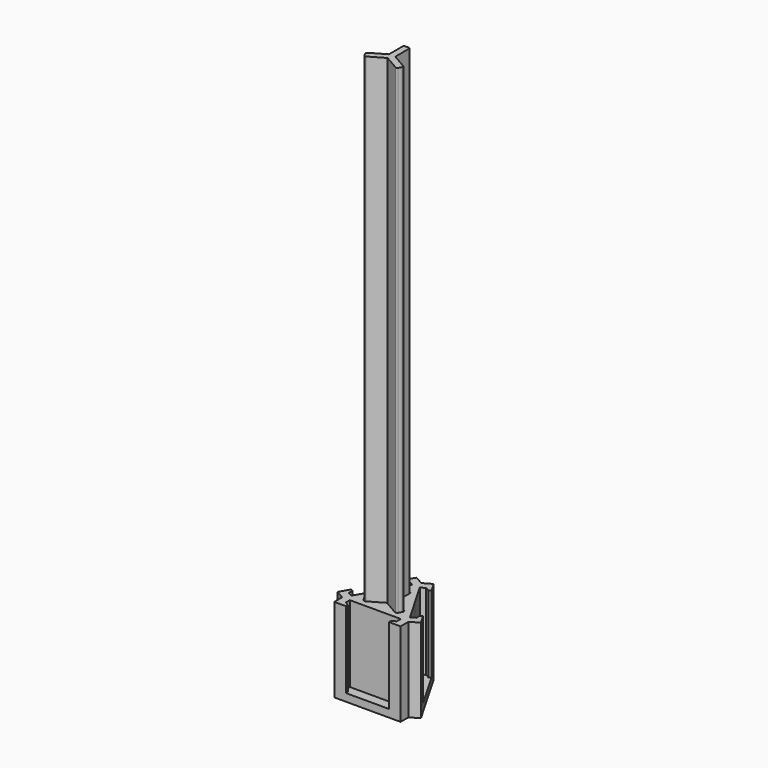
from build123d import *

# Parameters (mm, degrees)
F1_DEPTH      = 30
F3_DEPTH      = 3
F5_DEPTH      = 20
F5_DEPTH_BACK = 188
F6_OFFSET     = 0.3


with BuildPart() as f1:
    # F0 (on Top) → F1 (new body)
    with BuildSketch(Plane.XY):
        Polygon((-10, -7.5055534995), (0, -7.5055534995), (10, -7.5055534995), (10, -9.5055534995), (8.5, -10.3715789032), (8.5, -11.3715789032), (13, -11.3715789032), (13, -7.5055534995), (16.3480762114, -5.5725407976), (14.0980762114, -1.6754264805), (13.2320508076, -2.1754264805), (13.2320508076, -3.9074772881), (11.5, -4.9074772881), (6.5, 3.7527767497), (1.5, 12.4130307876), (3.2320508076, 13.4130307876), (4.7320508076, 12.5470053838), (5.5980762114, 13.0470053838), (3.3480762114, 16.9441197008), (0, 15.0111069989), (-3.3480762114, 16.9441197008), (-5.5980762114, 13.0470053838), (-4.7320508076, 12.5470053838), (-3.2320508076, 13.4130307876), (-1.5, 12.4130307876), (-6.5, 3.7527767497), (-11.5, -4.9074772881), (-13.2320508076, -3.9074772881), (-13.2320508076, -2.1754264805), (-14.0980762114, -1.6754264805), (-16.3480762114, -5.5725407976), (-13, -7.5055534995), (-13, -11.3715789032), (-8.5, -11.3715789032), (-8.5, -10.3715789032), (-10, -9.5055534995), align=None)
    extrude(amount=F1_DEPTH)

    # F2 (on face) → F3 (join)
    with BuildSketch(Plane(origin=(0, 0, 0), x_dir=(1, 0, 0), z_dir=(0, 0, -1))):
        Polygon((13, 11.3715789032), (-13, 11.3715789032), (-13, 7.5055534995), (-16.3480762114, 5.5725407976), (-3.3480762114, -16.9441197008), (0, -15.0111069989), (3.3480762114, -16.9441197008), (16.3480762114, 5.5725407976), (13, 7.5055534995), align=None)
    extrude(amount=F3_DEPTH)


with BuildPart() as f5:
    # F4 (on face) → F5 (new body, two sides)
    with BuildSketch(Plane.XY.offset(30)) as f5_sk:
        with BuildLine():
            Line((-1.25, 7.4), (-1.25, 0.7216878365))
            Line((-1.25, 0.7216878365), (-7.033587988, -2.6174682453))
            ThreePointArc((-7.033587988, -2.6174682453), (-7.3131434838, -2.9817920605), (-7.2532032303, -3.4370834875))
            Line((-7.2532032303, -3.4370834875), (-6.6032032303, -4.5629165125))
            ThreePointArc((-6.6032032303, -4.5629165125), (-6.2388794151, -4.8424720082), (-5.783587988, -4.7825317547))
            Line((-5.783587988, -4.7825317547), (0, -1.443375673))
            Line((0, -1.443375673), (5.783587988, -4.7825317547))
            ThreePointArc((5.783587988, -4.7825317547), (6.2388794151, -4.8424720082), (6.6032032303, -4.5629165125))
            Line((6.6032032303, -4.5629165125), (7.2532032303, -3.4370834875))
            ThreePointArc((7.2532032303, -3.4370834875), (7.3131434838, -2.9817920605), (7.033587988, -2.6174682453))
            Line((7.033587988, -2.6174682453), (1.25, 0.7216878365))
            Line((1.25, 0.7216878365), (1.25, 7.4))
            ThreePointArc((1.25, 7.4), (1.0742640687, 7.8242640687), (0.65, 8))
            Line((0.65, 8), (-0.65, 8))
            ThreePointArc((-0.65, 8), (-1.0742640687, 7.8242640687), (-1.25, 7.4))
        make_face()
    extrude(amount=-F5_DEPTH)
    extrude(f5_sk.sketch, amount=F5_DEPTH_BACK)


with BuildPart() as f1_1:
    add(f1.part)

    # F6: cut F5, made larger all round first
    f6_tool = offset(f5.part, amount=F6_OFFSET, kind=Kind.INTERSECTION, mode=Mode.PRIVATE)
    add(f6_tool, mode=Mode.SUBTRACT)


solid = Compound([f5.part, f1_1.part])
